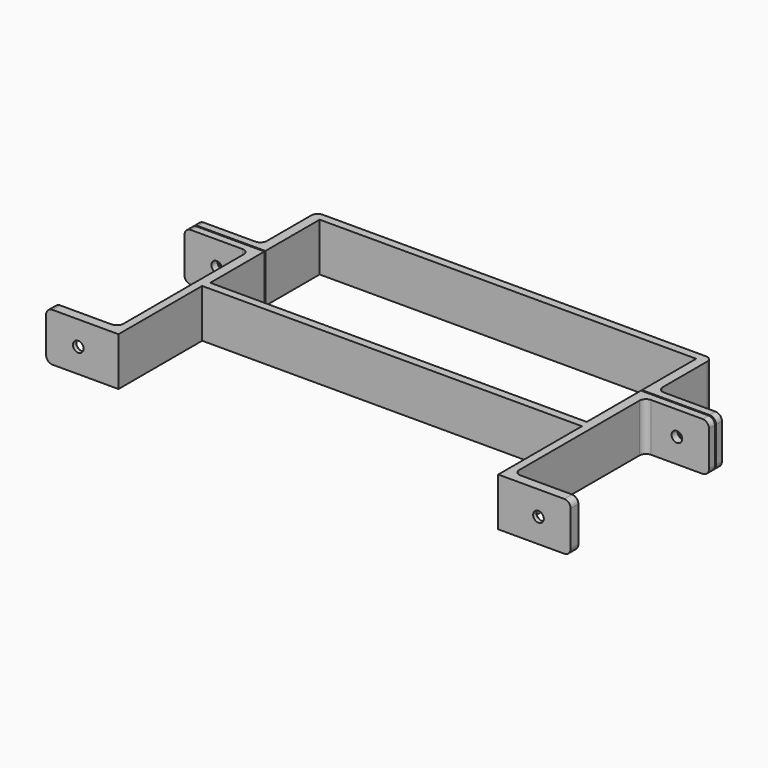
from build123d import *

# Parameters (mm, degrees)
F0_W            = 123
F0_H            = 47.5
F0_W_2          = 117
F0_H_2          = 42.5
F1_DEPTH        = 15
F3_W            = 2.5
F3_H            = 15
F4_DEPTH        = 32.5
F5_W            = 3
F5_H            = 15
F6_DEPTH        = 20
F7_W            = 3
F7_H            = 15
F8_DEPTH        = 20
F10_D           = 3.3
F10_DEPTH       = 5
F10_CSINK_D     = 6.72
F10_CSINK_ANGLE = 90
F10_TIP         = 0.9914200214
F12_D           = 3.3
F12_DEPTH       = 5
F12_CSINK_D     = 6.72
F12_CSINK_ANGLE = 90
F12_TIP         = 0.9914200214
F13_W           = 5
F13_H           = 15
F14_DEPTH       = 20
F16_D           = 3.3
F16_CSINK_D     = 6.72
F16_CSINK_ANGLE = 90
F17_W           = 5
F17_H           = 15
F18_DEPTH       = 20
F20_D           = 3.3
F20_CSINK_D     = 6.72
F20_CSINK_ANGLE = 90
F21_W           = 0.4
F21_H           = 15
F22_DEPTH       = 200
F23_R           = 2


with BuildPart() as f1:
    # F0 (on Top) → F1 (new body)
    with BuildSketch(Plane.XY):
        Rectangle(F0_W, F0_H)
        Rectangle(F0_W_2, F0_H_2, mode=Mode.SUBTRACT)
    extrude(amount=F1_DEPTH)

    # F3 (on face) → F4 (join)
    with BuildSketch(Plane.XZ.offset(23.75)):
        with Locations((-60.25, 7.5)):
            Rectangle(F3_W, F3_H)
        with Locations((60.25, 7.5)):
            Rectangle(F3_W, F3_H)
    extrude(amount=F4_DEPTH)

    # F5 (on face) → F6 (join)
    with BuildSketch(Plane(origin=(-61.5, 0, 0), x_dir=(0, -1, 0), z_dir=(-1, 0, 0))):
        with Locations((54.75, 7.5)):
            Rectangle(F5_W, F5_H)
    extrude(amount=F6_DEPTH)

    # F7 (on face) → F8 (join)
    with BuildSketch(Plane.YZ.offset(61.5)):
        with Locations((-54.75, 7.5)):
            Rectangle(F7_W, F7_H)
    extrude(amount=F8_DEPTH)

    # F10
    with Locations(Plane(origin=(0, -53.25, 0), x_dir=(-1, 0, 0), z_dir=(0, 1, 0))):
        with Locations((-71.5, 7.5)):
            CounterSinkHole(F10_D / 2, F10_CSINK_D / 2, depth=F10_DEPTH, counter_sink_angle=F10_CSINK_ANGLE)
            with Locations((0, 0, -(F10_DEPTH + F10_TIP / 2))):  # 118° drill point
                Cone(0, F10_D / 2, F10_TIP, mode=Mode.SUBTRACT)

    # F12
    with Locations(Plane(origin=(0, -53.25, 0), x_dir=(-1, 0, 0), z_dir=(0, 1, 0))):
        with Locations((71.5, 7.5)):
            CounterSinkHole(F12_D / 2, F12_CSINK_D / 2, depth=F12_DEPTH, counter_sink_angle=F12_CSINK_ANGLE)
            with Locations((0, 0, -(F12_DEPTH + F12_TIP / 2))):  # 118° drill point
                Cone(0, F12_D / 2, F12_TIP, mode=Mode.SUBTRACT)

    # F13 (on face) → F14 (join)
    with BuildSketch(Plane(origin=(-61.5, 0, 0), x_dir=(0, -1, 0), z_dir=(-1, 0, 0))):
        with Locations((0, 7.5)):
            Rectangle(F13_W, F13_H)
    extrude(amount=F14_DEPTH)

    # F16 (through all)
    with Locations(Plane(origin=(0, 2.5, 0), x_dir=(-1, 0, 0), z_dir=(0, 1, 0))):
        with Locations((71.5, 7.5)):
            CounterSinkHole(F16_D / 2, F16_CSINK_D / 2, counter_sink_angle=F16_CSINK_ANGLE)

    # F17 (on face) → F18 (join)
    with BuildSketch(Plane.YZ.offset(61.5)):
        with Locations((0, 7.5)):
            Rectangle(F17_W, F17_H)
    extrude(amount=F18_DEPTH)

    # F20 (through all)
    with Locations(Plane(origin=(0, 2.5, 0), x_dir=(-1, 0, 0), z_dir=(0, 1, 0))):
        with Locations((-71.5, 7.5)):
            CounterSinkHole(F20_D / 2, F20_CSINK_D / 2, counter_sink_angle=F20_CSINK_ANGLE)

    # F21 (on face) → F22 (cut)
    with BuildSketch(Plane.YZ.offset(81.5)):
        with Locations((0, 7.5)):
            Rectangle(F21_W, F21_H)
    extrude(amount=-F22_DEPTH, mode=Mode.SUBTRACT)

    # F23
    f23_edges = [f1.edges().sort_by_distance(p)[0] for p in [
        (-61.5, 23.75, 7.5),
        (-81.5, -1.35, 0),
        (-81.5, 1.35, 0),
        (-81.5, -54.75, 15),
        (81.5, -54.75, 0),
        (81.5, -1.35, 15),
        (81.5, 1.35, 15),
        (61.5, 23.75, 7.5),
        (-61.5, -53.25, 7.5),
        (61.5, -53.25, 7.5),
        (81.5, -1.35, 0),
        (81.5, 1.35, 0),
        (-81.5, -1.35, 15),
        (-81.5, 1.35, 15),
        (-61.5, 2.5, 7.5),
        (-61.5, -2.5, 7.5),
        (61.5, 2.5, 7.5),
        (61.5, -2.5, 7.5),
        (-81.5, -54.75, 0),
        (81.5, -54.75, 15),
    ]]
    fillet(f23_edges, radius=F23_R)


solid = f1.part
